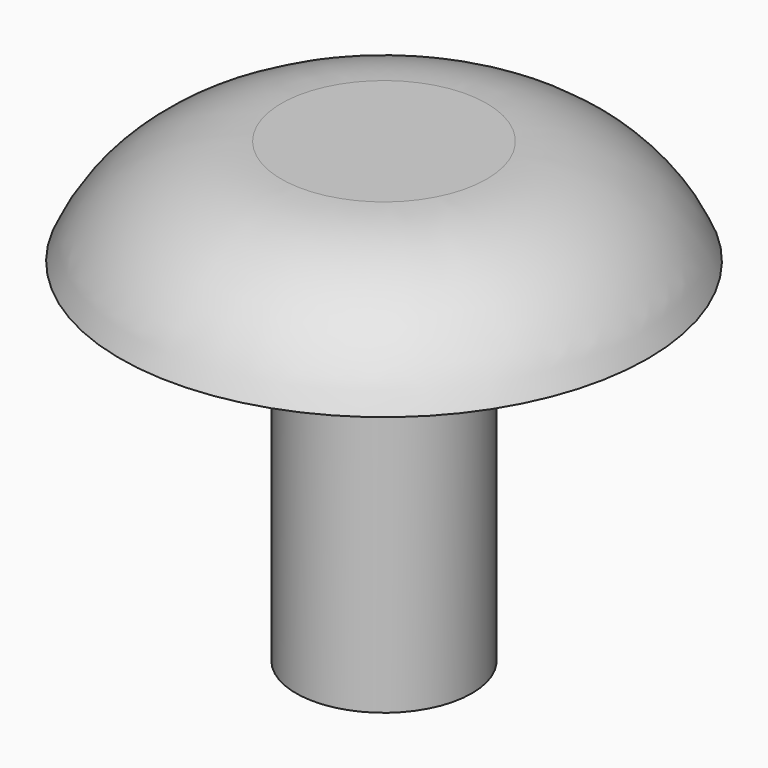
from build123d import *

# Parameters (mm, degrees)
F0_R     = 7.5
F1_DEPTH = 3
F3_R     = 2.5
F4_DEPTH = 10


# Not quite as in the source:
# - a fillet or chamfer that OpenCascade refuses, or shapes differently, is made with other operations: its cross-section is extruded or revolved along the edge and cut away or added


with BuildPart() as f1:
    # F0 (on Top) → F1 (new body)
    with BuildSketch(Plane.XY):
        Circle(F0_R)
    extrude(amount=F1_DEPTH)

    # F2: fillet of radius 5 on 1 edges, made by hand

    # F2_s1 → F2_t2 (revolve, cut)
    with BuildSketch(Plane.XZ):
        with BuildLine():
            ThreePointArc((7.5, 0), (5.6560370926, 2.1833001327), (2.917424305, 3))
            Line((2.917424305, 3), (7.5, 3))
            Line((7.5, 3), (7.5, 0))
        make_face()
    revolve(axis=Axis((0, 0, 3), (0, 0, 1)), mode=Mode.SUBTRACT)

    # F3 (on Top) → F4 (join)
    with BuildSketch(Plane.XY):
        Circle(F3_R)
    extrude(amount=-F4_DEPTH)


solid = f1.part
